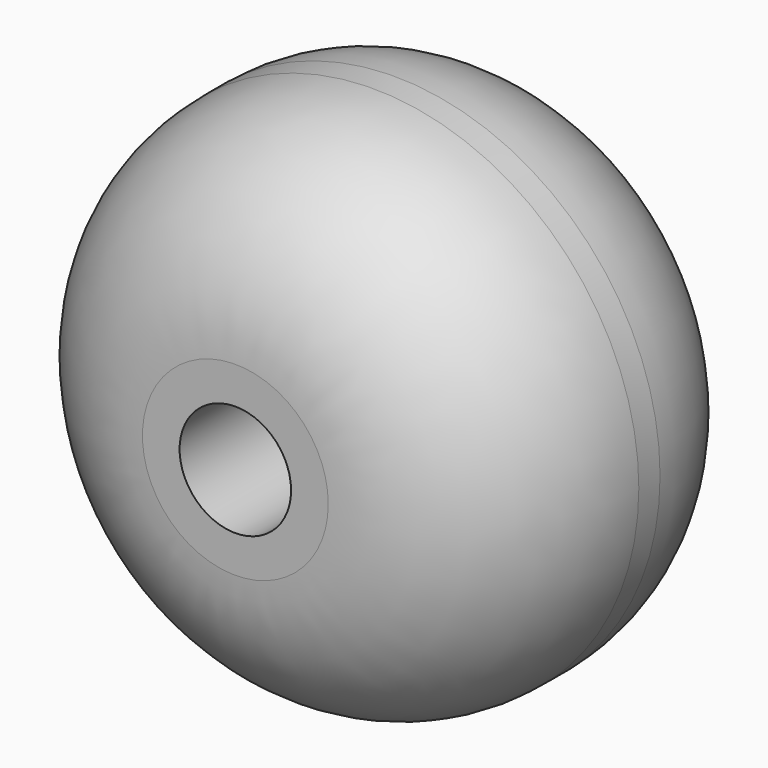
from build123d import *

# Parameters (mm, degrees)
F0_R          = 10
F0_R_2        = 2.1
F2_DEPTH      = 7
F2_DEPTH_BACK = 7
F3_R          = 6.5


# Not quite as in the source:
# - the program builds the solid bodies; features that only make, move or delete a surface that nothing else refers to are left out


with BuildPart() as f2:
    # F0 (on Front) → F2 (new body, two sides)
    with BuildSketch(Plane.XZ) as f2_sk:
        Circle(F0_R)
        Circle(F0_R_2, mode=Mode.SUBTRACT)
    extrude(amount=F2_DEPTH)
    extrude(f2_sk.sketch, amount=-F2_DEPTH_BACK)

    # F3
    f3_edges = [f2.edges().sort_by_distance(p)[0] for p in [
        (-10, -7, 0),
        (-10, 7, 0),
    ]]
    fillet(f3_edges, radius=F3_R)


solid = f2.part
